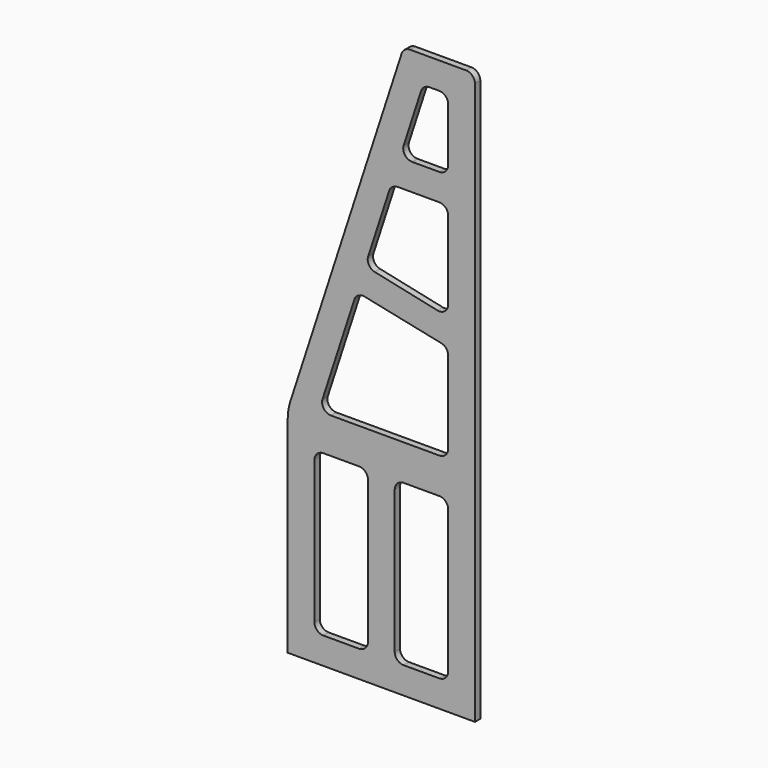
from build123d import *

# Parameters (mm, degrees)
F0_W     = 152.4
F0_H     = 457.2
F1_DEPTH = 19.05
F2_R     = 25.4
F4_R     = 152.4


# Not quite as in the source:
# - two fillets or chamfers of one size are made in one step


with BuildPart() as f1:
    # F0 (on Front) → F1 (new body)
    with BuildSketch(Plane.XZ):
        Polygon((266.7, -812.8), (266.7, 812.8), (63.5, 812.8), (-266.7, -203.2), (-266.7, -812.8), align=None)
        with Locations((-114.3, -508)):
            Rectangle(F0_W, F0_H, mode=Mode.SUBTRACT)
        with Locations((114.3, -508)):
            Rectangle(F0_W, F0_H, mode=Mode.SUBTRACT)
        Polygon((190.5, -177.8), (-178.3216873813, -177.8), (-79.2616873813, 127), (-69.7940460934, 156.1312039627), (190.5, 101.6), align=None, mode=Mode.SUBTRACT)
        Polygon((190.5, 457.2), (190.5, 228.6), (190.5, 177.8), (-46.2416873813, 228.6), (28.0533126187, 457.2), align=None, mode=Mode.SUBTRACT)
        Polygon((118.67604537, 736.6), (190.5, 736.6), (190.5, 533.4), (52.8183126187, 533.4), align=None, mode=Mode.SUBTRACT)
    extrude(amount=F1_DEPTH)

    # F2
    f2_edges = [f1.edges().sort_by_distance(p)[0] for p in [
        (28.053313, -9.525, 457.2),
        (-178.321687, -9.525, -177.8),
        (-190.5, -9.525, -279.4),
        (38.1, -9.525, -279.4),
        (-38.1, -9.525, -279.4),
        (190.5, -9.525, -279.4),
        (190.5, -9.525, 457.2),
        (190.5, -9.525, -177.8),
        (-190.5, -9.525, -736.6),
        (38.1, -9.525, -736.6),
        (-38.1, -9.525, -736.6),
        (190.5, -9.525, -736.6),
        (190.5, -9.525, 533.4),
        (266.7, -9.525, 812.8),
        (52.818313, -9.525, 533.4),
        (190.5, -9.525, 736.6),
        (118.676045, -9.525, 736.6),
        (190.5, -9.525, 177.8),
        (-46.241687, -9.525, 228.6),
        (-69.794046, -9.525, 156.131204),
        (190.5, -9.525, 101.6),
        (63.5, -9.525, 812.8),
    ]]
    fillet(f2_edges, radius=F2_R)

    # F4
    f4_edges = [f1.edges().sort_by_distance(p)[0] for p in [
        (-266.7, -9.525, -203.2),
    ]]
    fillet(f4_edges, radius=F4_R)


solid = f1.part
